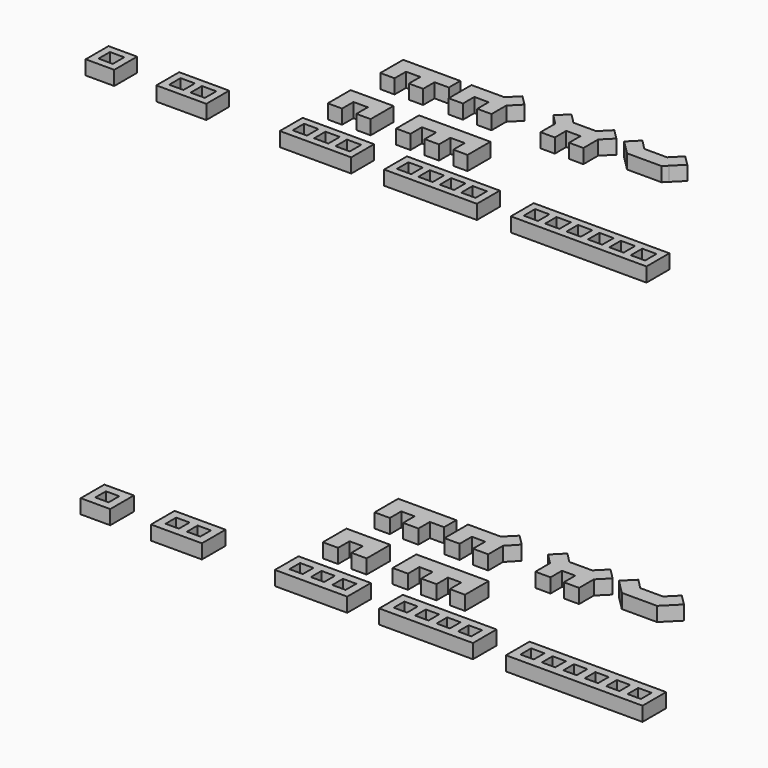
from build123d import *

# Parameters (mm, degrees)
F0_W     = 15
F0_H     = 6
F0_W_2   = 3
F0_H_2   = 3
F1_DEPTH = 3
F0_W_3   = 19.5
F0_W_4   = 10.5
F0_W_5   = 6
F0_W_6   = 28.5
F0_W_7   = 15.2
F0_H_3   = 6.2
F0_W_8   = 2.8
F0_H_4   = 2.8
F0_W_9   = 19.7
F0_W_10  = 10.7
F0_W_11  = 6.2
F0_W_12  = 28.7


# Not quite as in the source:
# - a feature names something its author has since deleted; it is built from what else it names


with BuildPart() as f1:
    # F0 (on Top) → F1 (new body)
    with BuildSketch(Plane.XY):
        with Locations((49.6419689059, 3)):
            Rectangle(F0_W, F0_H)
        with Locations((45.1419689059, 3)):
            Rectangle(F0_W_2, F0_H_2, mode=Mode.SUBTRACT)
        with Locations((49.6419689059, 3)):
            Rectangle(F0_W_2, F0_H_2, mode=Mode.SUBTRACT)
        with Locations((54.1419689059, 3)):
            Rectangle(F0_W_2, F0_H_2, mode=Mode.SUBTRACT)
    extrude(amount=F1_DEPTH)


with BuildPart() as f1b:
    # F0 (on Top) → F1, piece 2 (new body)
    with BuildSketch(Plane.XY):
        Polygon((42.1419689059, 18.5986374915), (42.1419689059, 12.5986374915), (45.1419689059, 12.5986374915), (45.1419689059, 15.5986374915), (48.1419689059, 15.5986374915), (48.1419689059, 12.5986374915), (51.1419689059, 12.5986374915), (51.1419689059, 18.5986374915), align=None)
    extrude(amount=F1_DEPTH)


with BuildPart() as f1c:
    # F0 (on Top) → F1, piece 3 (new body)
    with BuildSketch(Plane.XY):
        with Locations((73.803933382, 3)):
            Rectangle(F0_W_3, F0_H)
        with Locations((67.053933382, 3)):
            Rectangle(F0_W_2, F0_H_2, mode=Mode.SUBTRACT)
        with Locations((71.553933382, 3)):
            Rectangle(F0_W_2, F0_H_2, mode=Mode.SUBTRACT)
        with Locations((76.053933382, 3)):
            Rectangle(F0_W_2, F0_H_2, mode=Mode.SUBTRACT)
        with Locations((80.553933382, 3)):
            Rectangle(F0_W_2, F0_H_2, mode=Mode.SUBTRACT)
    extrude(amount=F1_DEPTH)


with BuildPart() as f1d:
    # F0 (on Top) → F1, piece 4 (new body)
    with BuildSketch(Plane.XY):
        with Locations((21.4413003027, 3)):
            Rectangle(F0_W_4, F0_H)
        with Locations((19.1913003027, 3)):
            Rectangle(F0_W_2, F0_H_2, mode=Mode.SUBTRACT)
        with Locations((23.6913003027, 3)):
            Rectangle(F0_W_2, F0_H_2, mode=Mode.SUBTRACT)
    extrude(amount=F1_DEPTH)


with BuildPart() as f1e:
    # F0 (on Top) → F1, piece 5 (new body)
    with BuildSketch(Plane.XY):
        with Locations((4.350495033, 3)):
            Rectangle(F0_W_5, F0_H)
        with Locations((4.350495033, 3)):
            Rectangle(F0_W_2, F0_H_2, mode=Mode.SUBTRACT)
    extrude(amount=F1_DEPTH)


with BuildPart() as f1f:
    # F0 (on Top) → F1, piece 6 (new body)
    with BuildSketch(Plane.XY):
        with Locations((104.9329522252, 3)):
            Rectangle(F0_W_6, F0_H)
        with Locations((93.6829522252, 3)):
            Rectangle(F0_W_2, F0_H_2, mode=Mode.SUBTRACT)
        with Locations((98.1829522252, 3)):
            Rectangle(F0_W_2, F0_H_2, mode=Mode.SUBTRACT)
        with Locations((102.6829522252, 3)):
            Rectangle(F0_W_2, F0_H_2, mode=Mode.SUBTRACT)
        with Locations((107.1829522252, 3)):
            Rectangle(F0_W_2, F0_H_2, mode=Mode.SUBTRACT)
        with Locations((111.6829522252, 3)):
            Rectangle(F0_W_2, F0_H_2, mode=Mode.SUBTRACT)
        with Locations((116.1829522252, 3)):
            Rectangle(F0_W_2, F0_H_2, mode=Mode.SUBTRACT)
    extrude(amount=F1_DEPTH)


with BuildPart() as f1g:
    # F0 (on Top) → F1, piece 7 (new body)
    with BuildSketch(Plane.XY):
        Polygon((71.5049424767, 18.5986374915), (56.5049424767, 18.5986374915), (56.5049424767, 12.5986374915), (59.5049424767, 12.5986374915), (59.5049424767, 15.5986374915), (62.5049424767, 15.5986374915), (62.5049424767, 12.5986374915), (65.5049424767, 12.5986374915), (65.5049424767, 15.5986374915), (68.5049424767, 15.5986374915), (68.5049424767, 12.5986374915), (71.5049424767, 12.5986374915), align=None)
    extrude(amount=F1_DEPTH)


with BuildPart() as f1h:
    # F0 (on Top) → F1, piece 8 (new body)
    with BuildSketch(Plane.XY):
        Polygon((51.1419689059, 32.3891406357), (42.1419689059, 32.3891406357), (42.1419689059, 26.3891406357), (45.1419689059, 26.3891406357), (45.1419689059, 29.3891406357), (48.1419689059, 29.3891406357), (48.1419689059, 26.3891406357), (51.1419689059, 26.3891406357), (51.1419689059, 29.3891406357), (54.1419689059, 29.3891406357), (54.1419689059, 32.3891406357), align=None)
    extrude(amount=F1_DEPTH)


with BuildPart() as f1i:
    # F0 (on Top) → F1, piece 9 (new body)
    with BuildSketch(Plane.XY):
        Polygon((63.3929424767, 32.3891406357), (56.5049424767, 32.3891406357), (56.5049424767, 26.3891406357), (59.5049424767, 26.3891406357), (59.5049424767, 29.3891406357), (62.5049424767, 29.3891406357), (62.5049424767, 26.3891406357), (65.5049424767, 26.3891406357), (65.5049424767, 30.2771406357), (65.5149424767, 30.2671406357), (67.6355831639, 32.3891406357), (65.5142628203, 34.5104609793), align=None)
    extrude(amount=F1_DEPTH)


with BuildPart() as f1j:
    # F0 (on Top) → F1, piece 10 (new body)
    with BuildSketch(Plane.XY):
        Polygon((82.6929488068, 32.3891406357), (77.9269488068, 32.3891406357), (75.8049488068, 34.5097813228), (73.6836284632, 32.3884609793), (75.8049488068, 30.2671406357), (75.8049488068, 26.3891406357), (78.8049488068, 26.3891406357), (78.8049488068, 29.3891406357), (81.8049488068, 29.3891406357), (81.8049488068, 26.3891406357), (84.8049488068, 26.3891406357), (84.8049488068, 30.2771406357), (84.8149488068, 30.2671406357), (86.9355894939, 32.3891406357), (84.8142691503, 34.5104609793), align=None)
    extrude(amount=F1_DEPTH)


with BuildPart() as f1k:
    # F0 (on Top) → F1, piece 11 (new body)
    with BuildSketch(Plane.XY):
        Polygon((97.5929551606, 32.3891406357), (92.8269551606, 32.3891406357), (90.7049551606, 34.5097813228), (88.5836348171, 32.3884609793), (90.7049551606, 30.2671406357), (91.5829551606, 29.3891406357), (93.7049551606, 29.3891406357), (96.7049551606, 29.3891406357), (98.8369551606, 29.3891406357), (99.7049551606, 30.2571406357), (99.7049551606, 30.2771406357), (99.7149551606, 30.2671406357), (101.8355958477, 32.3891406357), (99.7142755042, 34.5104609793), align=None)
        Polygon((99.7049551606, 30.2571406357), (99.7149551606, 30.2671406357), (99.7049551606, 30.2771406357), align=None)
    extrude(amount=F1_DEPTH)


with BuildPart() as f1l:
    # F0 (on Top) → F1, piece 12 (new body)
    with BuildSketch(Plane.XY):
        with Locations((146.5264474762, -119.1782675498)):
            Rectangle(F0_W_7, F0_H_3)
        with Locations((142.0264474762, -119.1782675498)):
            Rectangle(F0_W_8, F0_H_4, mode=Mode.SUBTRACT)
        with Locations((146.5264474762, -119.1782675498)):
            Rectangle(F0_W_8, F0_H_4, mode=Mode.SUBTRACT)
        with Locations((151.0264474762, -119.1782675498)):
            Rectangle(F0_W_8, F0_H_4, mode=Mode.SUBTRACT)
    extrude(amount=F1_DEPTH)


with BuildPart() as f1m:
    # F0 (on Top) → F1, piece 13 (new body)
    with BuildSketch(Plane.XY):
        Polygon((138.9264474762, -103.4796300584), (138.9264474762, -109.6796300584), (142.1264474762, -109.6796300584), (142.1264474762, -106.6796300584), (144.9264474762, -106.6796300584), (144.9264474762, -109.6796300584), (148.1264474762, -109.6796300584), (148.1264474762, -103.4796300584), align=None)
    extrude(amount=F1_DEPTH)


with BuildPart() as f1n:
    # F0 (on Top) → F1, piece 14 (new body)
    with BuildSketch(Plane.XY):
        with Locations((170.6884119523, -119.1782675498)):
            Rectangle(F0_W_9, F0_H_3)
        with Locations((163.9384119523, -119.1782675498)):
            Rectangle(F0_W_8, F0_H_4, mode=Mode.SUBTRACT)
        with Locations((168.4384119523, -119.1782675498)):
            Rectangle(F0_W_8, F0_H_4, mode=Mode.SUBTRACT)
        with Locations((172.9384119523, -119.1782675498)):
            Rectangle(F0_W_8, F0_H_4, mode=Mode.SUBTRACT)
        with Locations((177.4384119523, -119.1782675498)):
            Rectangle(F0_W_8, F0_H_4, mode=Mode.SUBTRACT)
    extrude(amount=F1_DEPTH)


with BuildPart() as f1o:
    # F0 (on Top) → F1, piece 15 (new body)
    with BuildSketch(Plane.XY):
        with Locations((118.325778873, -119.2782675498)):
            Rectangle(F0_W_10, F0_H_3)
        with Locations((116.075778873, -119.2782675498)):
            Rectangle(F0_W_8, F0_H_4, mode=Mode.SUBTRACT)
        with Locations((120.575778873, -119.2782675498)):
            Rectangle(F0_W_8, F0_H_4, mode=Mode.SUBTRACT)
    extrude(amount=F1_DEPTH)


with BuildPart() as f1p:
    # F0 (on Top) → F1, piece 16 (new body)
    with BuildSketch(Plane.XY):
        with Locations((101.2349736032, -119.1782675498)):
            Rectangle(F0_W_11, F0_H_3)
        with Locations((101.2349736032, -119.1782675498)):
            Rectangle(F0_W_8, F0_H_4, mode=Mode.SUBTRACT)
    extrude(amount=F1_DEPTH)


with BuildPart() as f1q:
    # F0 (on Top) → F1, piece 17 (new body)
    with BuildSketch(Plane.XY):
        with Locations((201.8174307955, -119.1782675498)):
            Rectangle(F0_W_12, F0_H_3)
        with Locations((190.5674307955, -119.1782675498)):
            Rectangle(F0_W_8, F0_H_4, mode=Mode.SUBTRACT)
        with Locations((195.0674307955, -119.1782675498)):
            Rectangle(F0_W_8, F0_H_4, mode=Mode.SUBTRACT)
        with Locations((199.5674307955, -119.1782675498)):
            Rectangle(F0_W_8, F0_H_4, mode=Mode.SUBTRACT)
        with Locations((204.0674307955, -119.1782675498)):
            Rectangle(F0_W_8, F0_H_4, mode=Mode.SUBTRACT)
        with Locations((208.5674307955, -119.1782675498)):
            Rectangle(F0_W_8, F0_H_4, mode=Mode.SUBTRACT)
        with Locations((213.0674307955, -119.1782675498)):
            Rectangle(F0_W_8, F0_H_4, mode=Mode.SUBTRACT)
    extrude(amount=F1_DEPTH)


with BuildPart() as f1r:
    # F0 (on Top) → F1, piece 18 (new body)
    with BuildSketch(Plane.XY):
        Polygon((168.797421047, -103.4796300584), (153.597421047, -103.4796300584), (153.597421047, -109.6796300584), (156.797421047, -109.6796300584), (156.797421047, -106.6796300584), (159.597421047, -106.6796300584), (159.597421047, -109.6796300584), (162.797421047, -109.6796300584), (162.797421047, -106.6796300584), (165.597421047, -106.6796300584), (165.597421047, -109.6796300584), (168.797421047, -109.6796300584), align=None)
    extrude(amount=F1_DEPTH)


with BuildPart() as f1s:
    # F0 (on Top) → F1, piece 19 (new body)
    with BuildSketch(Plane.XY):
        Polygon((148.1264474762, -89.8891269141), (138.9264474762, -89.8891269141), (138.9264474762, -96.0891269141), (142.1264474762, -96.0891269141), (142.1264474762, -93.0891269141), (144.9264474762, -93.0891269141), (144.9264474762, -96.0891269141), (148.1264474762, -96.0891269141), (148.1264474762, -93.0891269141), (151.1264474762, -93.0891269141), (151.1264474762, -89.8891269141), align=None)
    extrude(amount=F1_DEPTH)


with BuildPart() as f1t:
    # F0 (on Top) → F1, piece 20 (new body)
    with BuildSketch(Plane.XY):
        Polygon((160.477421047, -89.8891269141), (153.597421047, -89.8891269141), (153.597421047, -96.0891269141), (156.797421047, -96.0891269141), (156.797421047, -92.8891269141), (159.597421047, -92.8891269141), (159.597421047, -96.0891269141), (162.797421047, -96.0891269141), (162.797421047, -92.2091269141), (162.799421047, -92.2111269141), (164.9321937685, -89.9598375922), (162.6694520687, -87.6970958924), align=None)
    extrude(amount=F1_DEPTH)


with BuildPart() as f1u:
    # F0 (on Top) → F1, piece 21 (new body)
    with BuildSketch(Plane.XY):
        Polygon((179.686427377, -89.8891269141), (174.8929107766, -89.8891269141), (172.7601380552, -87.7563541926), (170.4973963554, -90.0190958924), (172.689427377, -92.2111269141), (172.689427377, -96.0891269141), (175.889427377, -96.0891269141), (175.889427377, -93.0891269141), (178.689427377, -93.0891269141), (178.689427377, -96.0891269141), (181.889427377, -96.0891269141), (181.889427377, -92.2109108595), (184.0818080691, -90.019229564), (181.819427377, -87.7561269141), align=None)
    extrude(amount=F1_DEPTH)


with BuildPart() as f1v:
    # F0 (on Top) → F1, piece 22 (new body)
    with BuildSketch(Plane.XY):
        Polygon((194.5503509232, -89.8776746451), (189.7814648614, -89.8776746451), (187.660144409, -87.7563541926), (185.3974027092, -90.0190958924), (187.5894337309, -92.2111269141), (188.4674337309, -93.0891269141), (195.8643820538, -93.0891269141), (196.8023292486, -92.1511797193), (196.8023292486, -92.1296529704), (196.813092623, -92.1404163449), (199.0051236447, -89.9483853232), (196.7423819449, -87.6856436234), align=None)
        Polygon((196.8023292486, -92.1511797193), (196.813092623, -92.1404163449), (196.8023292486, -92.1296529704), align=None)
    extrude(amount=F1_DEPTH)


solid = Compound([f1.part, f1b.part, f1c.part, f1d.part, f1e.part, f1f.part, f1g.part, f1h.part, f1i.part, f1j.part, f1k.part, f1l.part, f1m.part, f1n.part, f1o.part, f1p.part, f1q.part, f1r.part, f1s.part, f1t.part, f1u.part, f1v.part])
